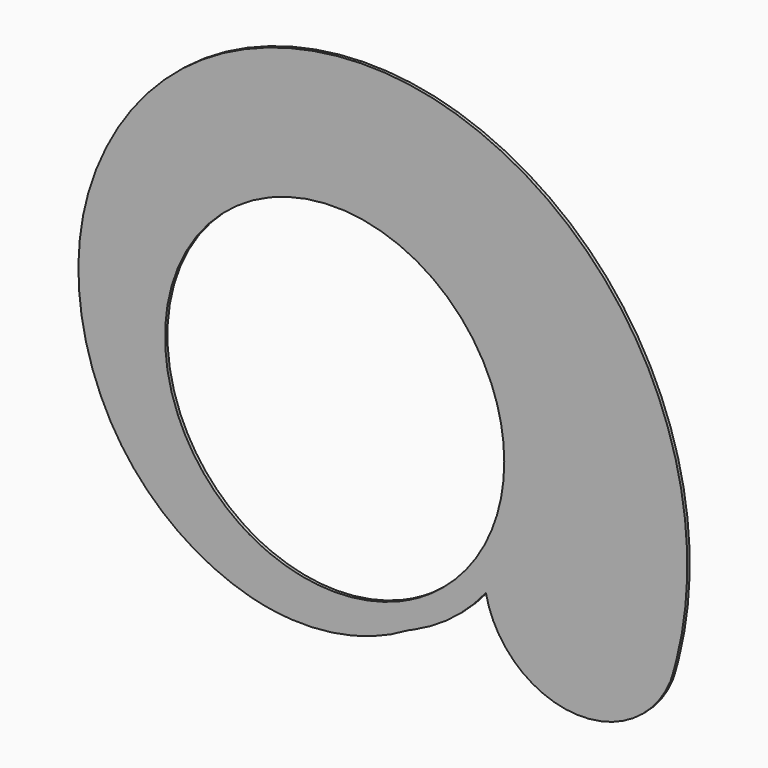
from build123d import *

# Parameters (mm, degrees)
F1_DEPTH = 3.175


with BuildPart() as f1:
    # F0 (on Front) → F1 (new body)
    with BuildSketch(Plane.XZ):
        with BuildLine():
            ThreePointArc((164.2657808805, 68.0411142745), (174.3836228557, 34.6870592545), (177.8, 0))
            ThreePointArc((177.8, 0), (174.3836228557, -34.6870592545), (164.2657808805, -68.0411142745))
            ThreePointArc((164.2657808805, -68.0411142745), (277.9531181005, -7.2739665138), (359.7319413837, -106.9217510028))
            ThreePointArc((359.7319413837, -106.9217510028), (359.3761364248, -115.4172186461), (358.3112136183, -123.8531837399))
            ThreePointArc((358.3112136183, -123.8531837399), (367.281161492, 8.8480312827), (328.531561761, 136.082228549))
            Line((328.531561761, 136.082228549), (164.2657808805, 68.0411142745))
        make_face()
        with BuildLine():
            ThreePointArc((68.0411142745, 164.2657808805), (125.723585695, 125.723585695), (164.2657808805, 68.0411142745))
            Line((164.2657808805, 68.0411142745), (328.531561761, 136.082228549))
            ThreePointArc((328.531561761, 136.082228549), (244.3258111618, 240.7675034736), (126.362069367, 305.0650216352))
            Line((126.362069367, 305.0650216352), (68.0411142745, 164.2657808805))
        make_face()
        with BuildLine():
            ThreePointArc((158.5532229762, -127.0870390081), (157.0041232469, -97.1378663495), (164.2657808805, -68.0411142745))
            ThreePointArc((164.2657808805, -68.0411142745), (137.7338592366, -112.4376450296), (99.5472631467, -147.32))
            ThreePointArc((99.5472631467, -147.32), (93.3013149914, -167.2172179653), (83.1243863135, -185.42))
            ThreePointArc((83.1243863135, -185.42), (124.3088906415, -160.740597571), (158.5532229762, -127.0870390081))
        make_face()
        with BuildLine():
            ThreePointArc((359.7319413837, -106.9217510028), (277.9531181005, -7.2739665138), (164.2657808805, -68.0411142745))
            Line((164.2657808805, -68.0411142745), (258.1319413837, -106.9217510028))
            Line((258.1319413837, -106.9217510028), (351.9981018868, -145.8023877311))
            ThreePointArc((351.9981018868, -145.8023877311), (355.3248382646, -134.8767336877), (358.3112136183, -123.8531837399))
            ThreePointArc((358.3112136183, -123.8531837399), (359.3761364248, -115.4172186461), (359.7319413837, -106.9217510028))
        make_face()
        with BuildLine():
            Line((258.1319413837, -106.9217510028), (164.2657808805, -68.0411142745))
            ThreePointArc((164.2657808805, -68.0411142745), (157.0041232469, -97.1378663495), (158.5532229762, -127.0870390081))
            ThreePointArc((158.5532229762, -127.0870390081), (248.3480567304, -208.0495691395), (351.9981018868, -145.8023877311))
            Line((351.9981018868, -145.8023877311), (258.1319413837, -106.9217510028))
        make_face()
        with BuildLine():
            ThreePointArc((-68.0411142745, 164.2657808805), (0, 177.8), (68.0411142745, 164.2657808805))
            Line((68.0411142745, 164.2657808805), (126.362069367, 305.0650216352))
            ThreePointArc((126.362069367, 305.0650216352), (2.514428483, 317.6217641107), (-116.6419101849, 281.5984815094))
            Line((-116.6419101849, 281.5984815094), (-68.0411142745, 164.2657808805))
        make_face()
        with BuildLine():
            ThreePointArc((83.1243863135, -185.42), (93.3013149914, -167.2172179653), (99.5472631467, -147.32))
            ThreePointArc((99.5472631467, -147.32), (84.2214695555, -156.5873049322), (68.0411142745, -164.2657808805))
            Line((68.0411142745, -164.2657808805), (77.7612734566, -187.7323210063))
            ThreePointArc((77.7612734566, -187.7323210063), (80.4511378852, -186.5954297752), (83.1243863135, -185.42))
        make_face()
        with BuildLine():
            ThreePointArc((-164.2657808805, 68.0411142745), (-125.723585695, 125.723585695), (-68.0411142745, 164.2657808805))
            Line((-68.0411142745, 164.2657808805), (-116.6419101849, 281.5984815094))
            ThreePointArc((-116.6419101849, 281.5984815094), (-204.8629851326, 208.4159123673), (-258.1319413837, 106.9217510028))
            Line((-258.1319413837, 106.9217510028), (-164.2657808805, 68.0411142745))
        make_face()
        with BuildLine():
            ThreePointArc((-164.2657808805, -68.0411142745), (-177.8, 0), (-164.2657808805, 68.0411142745))
            Line((-164.2657808805, 68.0411142745), (-258.1319413837, 106.9217510028))
            ThreePointArc((-258.1319413837, 106.9217510028), (-266.8448532831, 2.5095343628), (-234.6654012579, -97.2015918207))
            Line((-234.6654012579, -97.2015918207), (-164.2657808805, -68.0411142745))
        make_face()
        with BuildLine():
            ThreePointArc((-99.5472631467, -147.32), (-137.7338592366, -112.4376450296), (-164.2657808805, -68.0411142745))
            Line((-164.2657808805, -68.0411142745), (-234.6654012579, -97.2015918207))
            ThreePointArc((-234.6654012579, -97.2015918207), (-172.5099209033, -168.9661068295), (-87.4814326387, -211.1988611321))
            Line((-87.4814326387, -211.1988611321), (-79.0449703485, -190.8314394527))
            ThreePointArc((-79.0449703485, -190.8314394527), (-91.908148752, -170.3064913493), (-99.5472631467, -147.32))
        make_face()
        with BuildLine():
            Line((77.7612734566, -187.7323210063), (68.0411142745, -164.2657808805))
            ThreePointArc((68.0411142745, -164.2657808805), (34.6870592545, -174.3836228557), (0, -177.8))
            ThreePointArc((0, -177.8), (-34.6870592545, -174.3836228557), (-68.0411142745, -164.2657808805))
            Line((-68.0411142745, -164.2657808805), (-79.0449703485, -190.8314394527))
            ThreePointArc((-79.0449703485, -190.8314394527), (-63.7096435601, -206.143169746), (-45.4758683551, -217.8543086339))
            ThreePointArc((-45.4758683551, -217.8543086339), (18.4051257388, -212.0494957439), (77.7612734566, -187.7323210063))
        make_face()
        with BuildLine():
            ThreePointArc((-68.0411142745, -164.2657808805), (-84.2214695555, -156.5873049322), (-99.5472631467, -147.32))
            ThreePointArc((-99.5472631467, -147.32), (-91.908148752, -170.3064913493), (-79.0449703485, -190.8314394527))
            Line((-79.0449703485, -190.8314394527), (-68.0411142745, -164.2657808805))
        make_face()
        with BuildLine():
            ThreePointArc((-87.4814326387, -211.1988611321), (-66.6429296743, -215.563425688), (-45.4758683551, -217.8543086339))
            ThreePointArc((-45.4758683551, -217.8543086339), (-63.7096435601, -206.143169746), (-79.0449703485, -190.8314394527))
            Line((-79.0449703485, -190.8314394527), (-87.4814326387, -211.1988611321))
        make_face()
    extrude(amount=F1_DEPTH)


solid = f1.part
